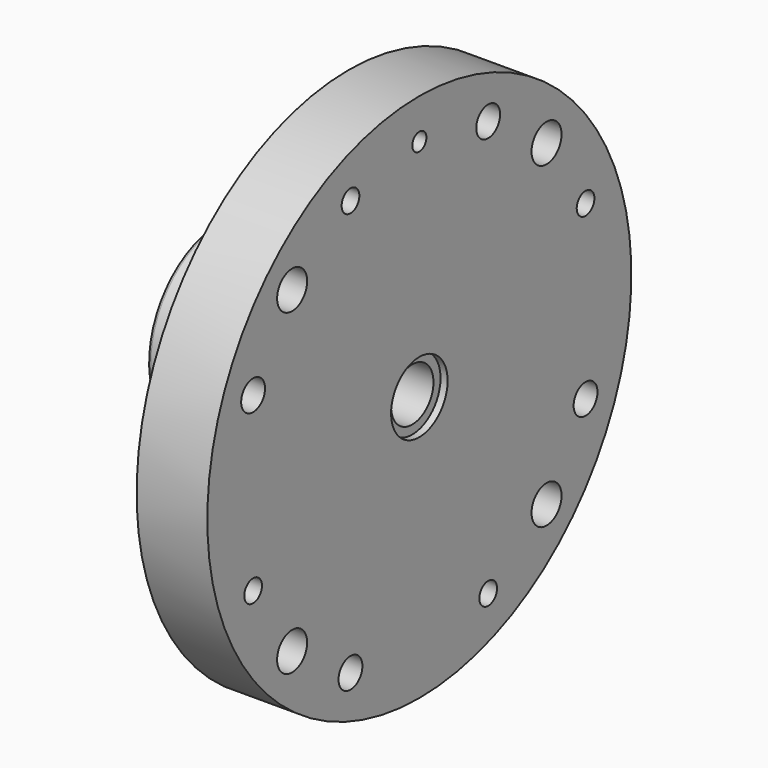
from build123d import *

# Parameters (mm, degrees)
F2_R             = 6.7437
F3_DEPTH         = 25.4
F3_COPIES_COUNT  = 4
F8_COPIES_COUNT  = 4
F11_COPIES_COUNT = 4
F12_R            = 3.175
F13_DEPTH        = 25.4


# Not quite as in the source:
# - a pattern or mirror of a feature is missing from the dataset's text; its kind, count and spacing are read off the source's solid


with BuildPart() as f1:
    # F0 (on Front) → F1 (revolve)
    with BuildSketch(Plane.XZ):
        with BuildLine():
            Line((-46.99, 30.4610814834), (-46.99, 0))
            Line((-46.99, 0), (25.4, 0))
            Line((25.4, 0), (25.4, 95.25))
            Line((25.4, 95.25), (0, 95.25))
            Line((0, 95.25), (0, 32.131))
            Line((0, 32.131), (-34.29, 32.131))
            Line((-34.29, 32.131), (-45.7643223608, 31.7303078338))
            ThreePointArc((-45.7643223608, 31.7303078338), (-46.6335615464, 31.3432976139), (-46.99, 30.4610814834))
        make_face()
    revolve(axis=Axis((-33.2340214019, 0, 0), (-1, 0, 0)))

    # F2 (on Right) → F3 (cut, through all)
    with BuildSketch(Plane.YZ):
        with Locations((57.15, 57.15)):
            Circle(F2_R)
    f3 = extrude(amount=F3_DEPTH, mode=Mode.SUBTRACT)

    # F3_copies: F3 ×4 about axis
    f3_copies_axis = Axis((0, 0, 0), (1, 0, 0))
    for i in range(1, F3_COPIES_COUNT):
        add(f3.rotate(f3_copies_axis, i * 360 / F3_COPIES_COUNT), mode=Mode.SUBTRACT)

    # F4 (on Front) → F5 (revolve, cut)
    with BuildSketch(Plane.XZ):
        Polygon((-38.0918026038, 9.525), (-43.815, 0), (25.4, 0), (25.4, 12.7), (22.86, 12.7), (22.86, 9.525), align=None)
    revolve(axis=Axis((25.4, 0, 0), (1, 0, 0)), mode=Mode.SUBTRACT)

    # F7 (on line) → F8 (revolve, cut)
    with BuildSketch(Plane(origin=(0, 0, 0), x_dir=(-1, 0, 0), z_dir=(0, 0.9238795325, -0.3826834324))):
        Polygon((-25.4, 80.8228), (0, 80.8228), (0, 84.3915), (-15.494, 84.3915), (-15.494, 86.1822), (-25.4, 86.1822), align=None)
    f8 = revolve(axis=Axis((19.0941668783, 30.9295465174, 74.6705306803), (-1, 0, 0)), mode=Mode.SUBTRACT)

    # F8_copies: F8 ×4 about axis
    f8_copies_axis = Axis((0, 0, 0), (1, 0, 0))
    for i in range(1, F8_COPIES_COUNT):
        add(f8.rotate(f8_copies_axis, i * 360 / F8_COPIES_COUNT), mode=Mode.SUBTRACT)

    # F10 (on line) → F11 (revolve, cut)
    with BuildSketch(Plane(origin=(0, 0, 0), x_dir=(-1, 0, 0), z_dir=(0, 0.9238795325, 0.3826834324))):
        Polygon((-25.4, 84.79155), (-25.4, 80.8228), (-2.9182675346, 80.8228), (-4.826, 83.9978), (-7.9248, 83.9978), (-7.9248, 84.79155), align=None)
    f11 = revolve(axis=Axis((19.9955312124, -30.9295465174, 74.6705306803), (-1, 0, 0)), mode=Mode.SUBTRACT)

    # F11_copies: F11 ×4 about axis
    f11_copies_axis = Axis((0, 0, 0), (1, 0, 0))
    for i in range(1, F11_COPIES_COUNT):
        add(f11.rotate(f11_copies_axis, i * 360 / F11_COPIES_COUNT), mode=Mode.SUBTRACT)

    # F12 (on Right) → F13 (cut, through all)
    with BuildSketch(Plane.YZ):
        with Locations((0, 80.8228)):
            Circle(F12_R)
    extrude(amount=F13_DEPTH, mode=Mode.SUBTRACT)


solid = f1.part
